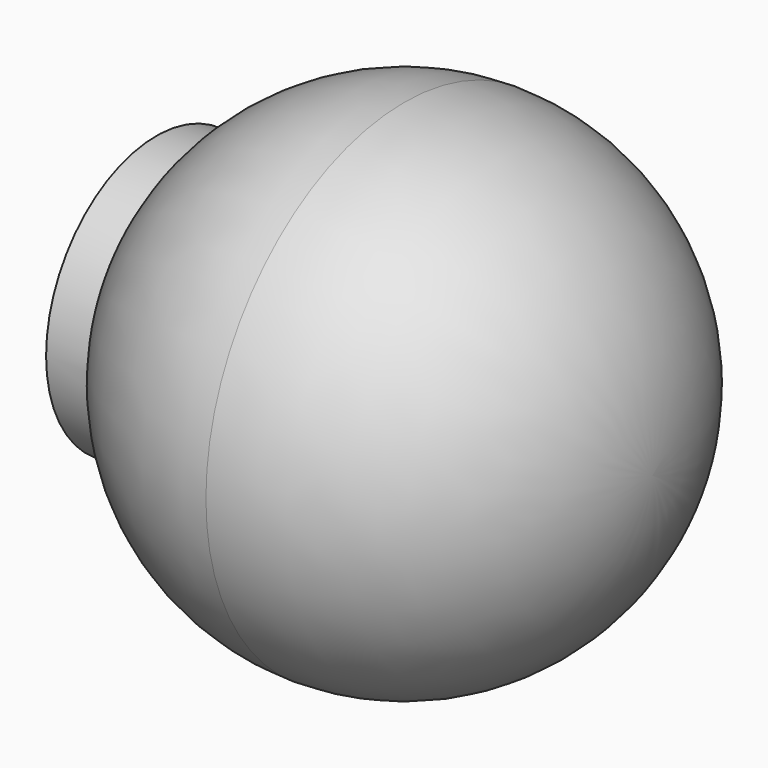
from build123d import *

# Parameters (mm, degrees)
F0_R     = 57.15
F1_DEPTH = 57.15
F2_R     = 57.15
F3_DEPTH = 57.15
F4_R     = 57.14999
F5_R     = 57.14999
F6_R     = 31.75
F7_DEPTH = 57.15


# Not quite as in the source:
# - a fillet or chamfer is up to 0.001 mm smaller than in the source, because OpenCascade refuses the exact size


with BuildPart() as f1:
    # F0 (on Right) → F1 (new body)
    with BuildSketch(Plane.YZ):
        Circle(F0_R)
    extrude(amount=F1_DEPTH)

    # F2 (on face) → F3 (join)
    with BuildSketch(Plane(origin=(0, 0, 0), x_dir=(0, -1, 0), z_dir=(-1, 0, 0))):
        Circle(F2_R)
    extrude(amount=F3_DEPTH)

    # F4 (radius 57.15 in the source; OpenCascade refuses exactly that, so slightly less here)
    f4_edges = [f1.edges().sort_by_distance(p)[0] for p in [
        (-57.15, 57.15, 0),
    ]]
    fillet(f4_edges, radius=F4_R)

    # F5 (radius 57.15 in the source; OpenCascade refuses exactly that, so slightly less here)
    f5_edges = [f1.edges().sort_by_distance(p)[0] for p in [
        (57.15, -57.15, 0),
    ]]
    fillet(f5_edges, radius=F5_R)

    # F6 (on face) → F7 (join)
    with BuildSketch(Plane(origin=(0, 0, 0), x_dir=(0, -1, 0), z_dir=(-1, 0, 0))):
        Circle(F6_R)
    extrude(amount=F7_DEPTH)


solid = f1.part
